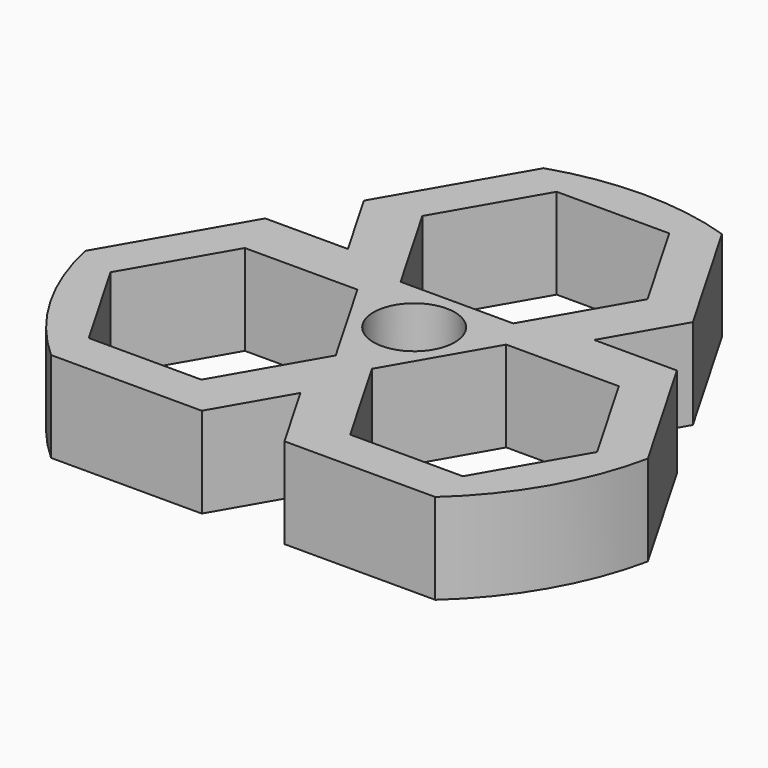
from build123d import *

# Parameters (mm, degrees)
F0_R     = 3.5
F1_DEPTH = 7.8


# Not quite as in the source:
# - the program builds the solid bodies; features that only make, move or delete a surface that nothing else refers to are left out


with BuildPart() as f1:
    # F0 (on Top) → F1 (new body)
    with BuildSketch(Plane.XY):
        with BuildLine():
            ThreePointArc((16.5459263903, -18.417339772), (21.4411884767, -12.3790759388), (24.2228473078, -5.1205226972))
            Line((24.2228473078, -5.1205226972), (17.7308233658, 6.1239926144))
            Line((17.7308233658, 6.1239926144), (10.6070663534, 6.1239926144))
            Line((10.6070663534, 6.1239926144), (14.1689448596, 12.2933471575))
            Line((14.1689448596, 12.2933471575), (7.6769209175, 23.5378624692))
            ThreePointArc((7.6769209175, 23.5378624692), (0, 24.7581518775), (-7.6769209175, 23.5378624692))
            Line((-7.6769209175, 23.5378624692), (-14.1689448596, 12.2933471575))
            Line((-14.1689448596, 12.2933471575), (-10.6070663534, 6.1239926144))
            Line((-10.6070663534, 6.1239926144), (-17.7308233658, 6.1239926144))
            Line((-17.7308233658, 6.1239926144), (-24.2228473078, -5.1205226972))
            ThreePointArc((-24.2228473078, -5.1205226972), (-21.4411884767, -12.3790759388), (-16.5459263903, -18.417339772))
            Line((-16.5459263903, -18.417339772), (-3.5618785062, -18.417339772))
            Line((-3.5618785062, -18.417339772), (0, -12.2479852289))
            Line((0, -12.2479852289), (3.5618785062, -18.417339772))
            Line((3.5618785062, -18.417339772), (16.5459263903, -18.417339772))
        make_face()
        Polygon((-6.408587988, -14.9), (-16.1080725104, -14.9), (-20.9578147716, -6.5), (-16.1080725104, 1.9), (-6.408587988, 1.9), (-1.5588457268, -6.5), align=None, mode=Mode.SUBTRACT)
        Polygon((16.1080725104, 1.9), (20.9578147716, -6.5), (16.1080725104, -14.9), (6.408587988, -14.9), (1.5588457268, -6.5), (6.408587988, 1.9), align=None, mode=Mode.SUBTRACT)
        Circle(F0_R, mode=Mode.SUBTRACT)
        Polygon((9.6994845224, 13), (4.8497422612, 4.6), (-4.8497422612, 4.6), (-9.6994845224, 13), (-4.8497422612, 21.4), (4.8497422612, 21.4), align=None, mode=Mode.SUBTRACT)
    extrude(amount=F1_DEPTH)


solid = f1.part
